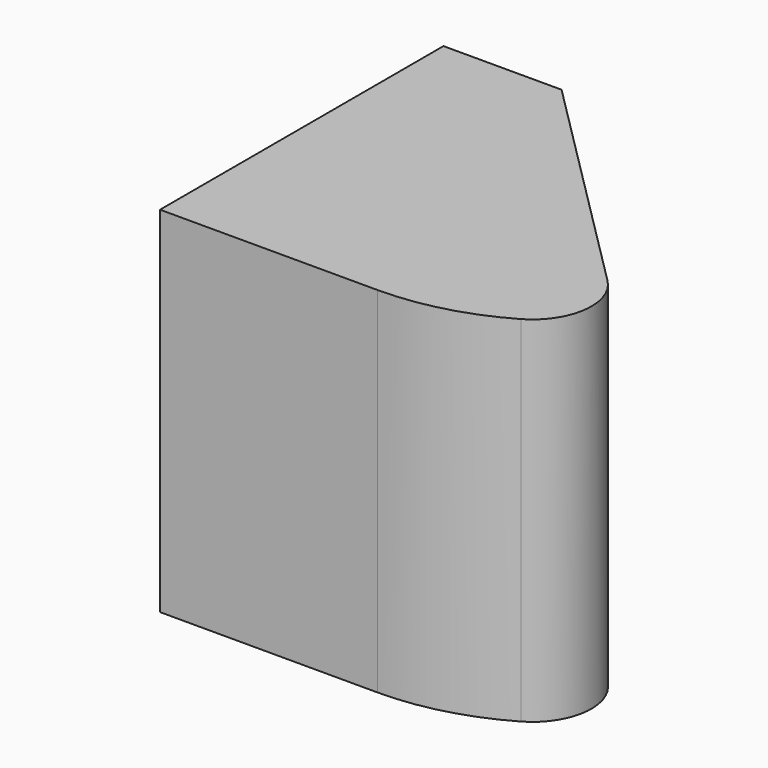
from build123d import *

# Parameters (mm, degrees)
F1_DEPTH    = 300
F2_T1_DEPTH = 778.5765609082
F3_R        = 50
F5_R        = 35
F6_DEPTH    = 250


# Not quite as in the source:
# - a fillet or chamfer that OpenCascade refuses, or shapes differently, is made with other operations: its cross-section is extruded or revolved along the edge and cut away or added


with BuildPart() as f1:
    # F0 (on Top) → F1 (new body)
    with BuildSketch(Plane.XY):
        Polygon((0, 300), (0, 0), (280, 0), (333.3452377916, 66.6547622084), (100, 300), align=None)
    extrude(amount=-F1_DEPTH)

    # F2: fillet of radius 200 on 1 edges, made by hand

    # F2_s2 → F2_t1 (cut)
    with BuildSketch(Plane.XY.offset(-539.2882804541)):
        with BuildLine():
            ThreePointArc((184.2846878184, 0), (265.9270556236, 17.4225540239), (333.3452377916, 66.6547622084))
            Line((333.3452377916, 66.6547622084), (280, 0))
            Line((280, 0), (184.2846878184, 0))
        make_face()
    extrude(amount=F2_T1_DEPTH, mode=Mode.SUBTRACT)

    # F3
    f3_edges = [f1.edges().sort_by_distance(p)[0] for p in [
        (333.345238, 66.654762, -150),
    ]]
    fillet(f3_edges, radius=F3_R)

    # F5 (on face) → F6 (cut)
    with BuildSketch(Plane(origin=(-114.9066664678, 53.581858547, 0), x_dir=(-0.4226182617, -0.906307787, 0), z_dir=(-0.906307787, 0.4226182617, 0))):
        with Locations((-171.892336111, -150)):
            Circle(F5_R)
    extrude(amount=-F6_DEPTH, mode=Mode.SUBTRACT)


solid = f1.part
